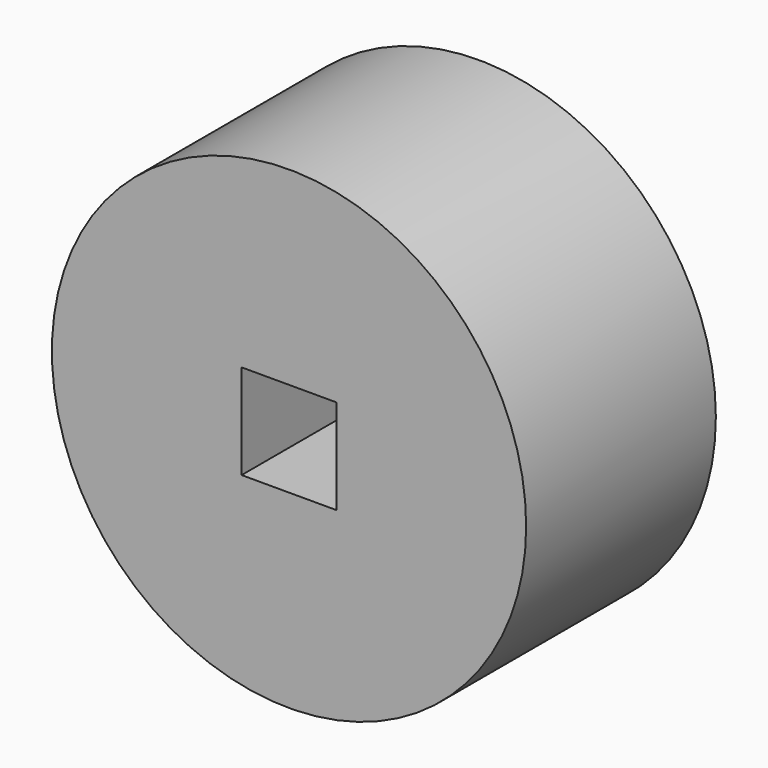
from build123d import *

# Parameters (mm, degrees)
F0_R     = 25
F0_W     = 10
F0_H     = 10
F2_DEPTH = 25


# Not quite as in the source:
# - the program builds the solid bodies; features that only make, move or delete a surface that nothing else refers to are left out


with BuildPart() as f2:
    # F0 (on Front) → F2 (new body)
    with BuildSketch(Plane.XZ):
        Circle(F0_R)
        Rectangle(F0_W, F0_H, mode=Mode.SUBTRACT)
    extrude(amount=F2_DEPTH)


solid = f2.part
